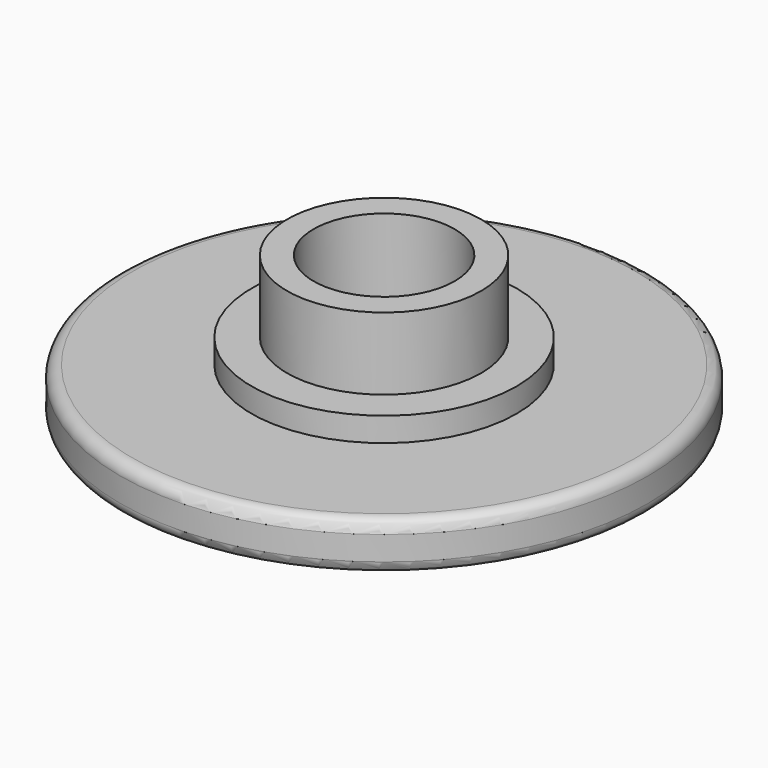
from build123d import *

# Parameters (mm, degrees)
F0_R         = 10.95
F0_R_2       = 0.069
F3_DEPTH     = 2
F1_R         = 5.5
F4_DEPTH     = 3
F2_R         = 4.025
F5_DEPTH     = 6
F6_R         = 0.5
F7_R         = 2.9249999207
F8_DEPTH     = 4
F9_TEXT_SIZE = 9.5471529575
F10_DEPTH    = 1


# Not quite as in the source:
# - Text() gives the source's letters only with a copy of the font that has no kerning and outlines rounded to 1/6400 em; it was checked with that copy


with BuildPart() as f3:
    # F0 (on Top) → F3 (new body)
    with BuildSketch(Plane.XY):
        Circle(F0_R)
        Circle(F0_R_2, mode=Mode.SUBTRACT)
    extrude(amount=F3_DEPTH)

    # F1 (on Top) → F4 (join)
    with BuildSketch(Plane.XY):
        Circle(F1_R)
    extrude(amount=F4_DEPTH)

    # F2 (on Top) → F5 (join)
    with BuildSketch(Plane.XY):
        Circle(F2_R)
    extrude(amount=F5_DEPTH)

    # F6
    f6_edges = [f3.edges().sort_by_distance(p)[0] for p in [
        (10.95, 0, 1),
        (-10.95, 0, 0),
        (-10.95, 0, 2),
    ]]
    fillet(f6_edges, radius=F6_R)

    # F7 (on face) → F8 (cut)
    with BuildSketch(Plane.XY.offset(6)):
        Circle(F7_R)
    extrude(amount=-F8_DEPTH, mode=Mode.SUBTRACT)

    # F9 (on face) → F10 (cut)
    with BuildSketch(Plane(origin=(0, 0, 0), x_dir=(1, 0, 0), z_dir=(0, 0, -1))):
        with Locations((-9.8813027143, -2.966437256)):
            Text('Nick', F9_TEXT_SIZE, font='Open Sans', text_align=(TextAlign.LEFT, TextAlign.BOTTOM))
    extrude(amount=-F10_DEPTH, mode=Mode.SUBTRACT)


solid = f3.part
